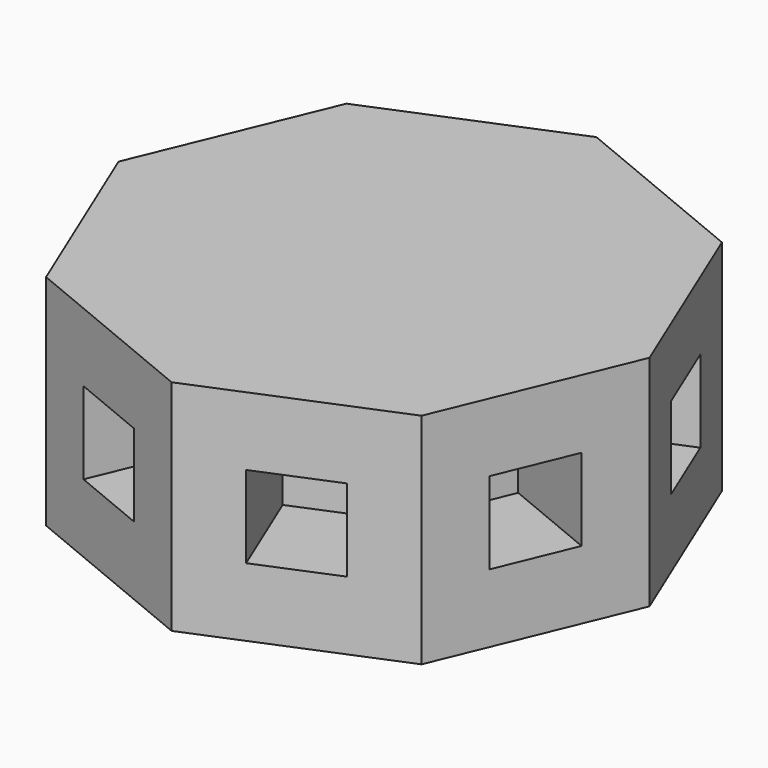
from build123d import *

# Parameters (mm, degrees)
F1_DEPTH        = 16
F2_W            = 12
F2_H            = 12
F4_DEPTH        = 15
F4_COPIES_COUNT = 8
F5_W            = 32
F5_H            = 32
F6_DEPTH        = 38.627


# Not quite as in the source:
# - a pattern or mirror of a feature is missing from the dataset's text; its kind, count and spacing are read off the source's solid


with BuildPart() as f1:
    # F0 (on Top) → F1 (new body, symmetric)
    with BuildSketch(Plane.XY):
        Polygon((-27.4452890516, 27.4452890516), (-38.8135, 0), (-27.4452890516, -27.4452890516), (0, -38.8135), (27.4452890516, -27.4452890516), (38.8135, 0), (27.4452890516, 27.4452890516), (0, 38.8135), align=None)
    extrude(amount=F1_DEPTH, both=True)

    # F2 (on face) → F4 (cut)
    with BuildSketch(Plane(origin=(-13.7226445258, -33.1293945258, 0), x_dir=(0.9238795325, -0.3826834324, 0), z_dir=(-0.3826834324, -0.9238795325, 0))):
        Rectangle(F2_W, F2_H)
    f4 = extrude(amount=-F4_DEPTH, mode=Mode.SUBTRACT)

    # F4_copies: F4 ×8 about axis
    f4_copies_axis = Axis((0, 0, 0), (0, 0, 1))
    for i in range(1, F4_COPIES_COUNT):
        add(f4.rotate(f4_copies_axis, i * 360 / F4_COPIES_COUNT), mode=Mode.SUBTRACT)


with BuildPart() as f6:
    # F5 (on Top) → F6 (new body, symmetric)
    with BuildSketch(Plane.XY):
        Rectangle(F5_W, F5_H)
    extrude(amount=F6_DEPTH, both=True)


solid = f1.part
